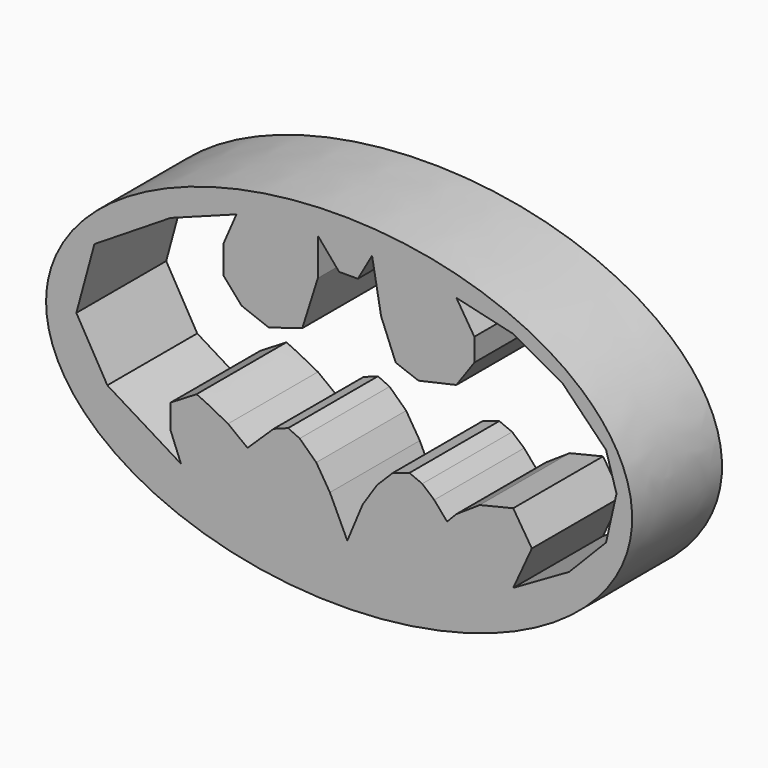
from build123d import *

# Parameters (mm, degrees)
F1_DEPTH = 25.4


with BuildPart() as f1:
    # F0 (on Front) → F1 (new body)
    with BuildSketch(Plane.XZ):
        with BuildLine():
            add(Edge.make_bspline(
                [(-66.2678331137, 0), (-66.2678331137, -67.3857780636), (33.1339165568, -33.6928890318), (132.5356662273, 0), (33.1339165568, 33.6928890318), (-66.2678331137, 67.3857780636), (-66.2678331137, 0)],
                knots=[0, 0, 0, 2.0943951024, 2.0943951024, 4.1887902048, 4.1887902048, 6.2831853072, 6.2831853072, 6.2831853072], degree=2, weights=[1, 0.5, 1, 0.5, 1, 0.5, 1]))
        make_face()
        with BuildLine():
            add(Edge.make_bspline(
                [(-38.1069518626, 25.8426479995), (-33.1428280721, 27.69202739), (-28.1787042816, 29.5414067805), (-23.2145804912, 31.390786171)],
                knots=[0, 0, 0, 0, 15.892279957, 15.892279957, 15.892279957, 15.892279957], degree=3))
            add(Edge.make_bspline(
                [(-23.2145804912, 31.390786171), (-24.1879379998, 29.152063032), (-25.1612955083, 26.913339893), (-26.1346530169, 24.6746167541)],
                knots=[0, 0, 0, 0, 7.3235070282, 7.3235070282, 7.3235070282, 7.3235070282], degree=3))
            add(Edge.make_bspline(
                [(-26.1346530169, 24.6746167541), (-26.1346530169, 22.5332298627), (-26.1346530169, 20.3918429712), (-26.1346530169, 18.2504560798)],
                knots=[0, 0, 0, 0, 6.4241606742, 6.4241606742, 6.4241606742, 6.4241606742], degree=3))
            add(Edge.make_bspline(
                [(-26.1346530169, 18.2504560798), (-24.7719523807, 16.6930838798), (-23.4092517445, 15.1357116799), (-22.0465511084, 13.5783394799)],
                knots=[0, 0, 0, 0, 6.2081600123, 6.2081600123, 6.2081600123, 6.2081600123], degree=3))
            add(Edge.make_bspline(
                [(-22.0465511084, 13.5783394799), (-20.0024998436, 12.7996532246), (-17.9584485789, 12.0209669694), (-15.9143973142, 11.2422807142)],
                knots=[0, 0, 0, 0, 6.5620485149, 6.5620485149, 6.5620485149, 6.5620485149], degree=3))
            add(Edge.make_bspline(
                [(-15.9143973142, 11.2422807142), (-13.3836676056, 12.0209669694), (-10.852937897, 12.7996532246), (-8.3222081885, 13.5783394799)],
                knots=[0, 0, 0, 0, 7.9434568216, 7.9434568216, 7.9434568216, 7.9434568216], degree=3))
            add(Edge.make_bspline(
                [(-8.3222081885, 13.5783394799), (-7.1541789609, 17.2770985713), (-5.9861497333, 20.9758576627), (-4.8181205057, 24.6746167541)],
                knots=[0, 0, 0, 0, 11.6364083735, 11.6364083735, 11.6364083735, 11.6364083735], degree=3))
            add(Edge.make_bspline(
                [(-4.8181205057, 24.6746167541), (-4.8181205057, 27.4973536531), (-4.8181205057, 30.3200905522), (-4.8181205057, 33.1428274512)],
                knots=[0, 0, 0, 0, 8.4682106972, 8.4682106972, 8.4682106972, 8.4682106972], degree=3))
            add(Edge.make_bspline(
                [(-4.8181205057, 33.1428274512), (-3.2120803371, 31.2610028519), (-1.6060401686, 29.3791782525), (0, 27.4973536531)],
                knots=[0, 0, 0, 0, 7.4219714101, 7.4219714101, 7.4219714101, 7.4219714101], degree=3))
            add(Edge.make_bspline(
                [(4.2341067456, 27.4973536531), (2.8227378304, 27.4973536531), (1.4113689152, 27.4973536531), (0, 27.4973536531)],
                knots=[0, 0, 0, 0, 4.2341067456, 4.2341067456, 4.2341067456, 4.2341067456], degree=3))
            add(Edge.make_bspline(
                [(4.2341067456, 27.4973536531), (5.3048000361, 29.3791782525), (6.3754933265, 31.2610028519), (7.446186617, 33.1428274512)],
                knots=[0, 0, 0, 0, 6.4952930269, 6.4952930269, 6.4952930269, 6.4952930269], degree=3))
            add(Edge.make_bspline(
                [(7.446186617, 33.1428274512), (8.1275366247, 29.3467330436), (8.8088866323, 25.550638636), (9.49023664, 21.7545442283)],
                knots=[0, 0, 0, 0, 11.570269455, 11.570269455, 11.570269455, 11.570269455], degree=3))
            add(Edge.make_bspline(
                [(9.49023664, 21.7545442283), (10.5910257747, 19.0358640005), (11.6918149094, 16.3171837727), (12.7926040441, 13.5985035449)],
                knots=[0, 0, 0, 0, 8.7992403138, 8.7992403138, 8.7992403138, 8.7992403138], degree=3))
            add(Edge.make_bspline(
                [(12.7926040441, 13.5985035449), (14.5068193475, 12.9556724181), (16.221034651, 12.3128412912), (17.9352499545, 11.6700101644)],
                knots=[0, 0, 0, 0, 5.4923486487, 5.4923486487, 5.4923486487, 5.4923486487], degree=3))
            add(Edge.make_bspline(
                [(17.9352499545, 11.6700101644), (20.7922750463, 12.3128412912), (23.6493001382, 12.9556724181), (26.50632523, 13.5985035449)],
                knots=[0, 0, 0, 0, 8.7853524743, 8.7853524743, 8.7853524743, 8.7853524743], degree=3))
            add(Edge.make_bspline(
                [(26.50632523, 13.5985035449), (27.8634124746, 15.5269963046), (29.2204997192, 17.4554890643), (30.5775869638, 19.3839818239)],
                knots=[0, 0, 0, 0, 7.0743855579, 7.0743855579, 7.0743855579, 7.0743855579], degree=3))
            add(Edge.make_bspline(
                [(30.5775869638, 19.3839818239), (30.5775869638, 21.0981971274), (30.5775869638, 22.8124124308), (30.5775869638, 24.5266277343)],
                knots=[0, 0, 0, 0, 5.1426459104, 5.1426459104, 5.1426459104, 5.1426459104], degree=3))
            add(Edge.make_bspline(
                [(30.5775869638, 24.5266277343), (29.2204997192, 26.6693979502), (27.8634124746, 28.812168166), (26.50632523, 30.9549383819)],
                knots=[0, 0, 0, 0, 7.6090965224, 7.6090965224, 7.6090965224, 7.6090965224], degree=3))
            add(Edge.make_bspline(
                [(26.50632523, 30.9549383819), (30.7918662826, 29.9549791962), (35.0774073352, 28.9550200105), (39.3629483879, 27.9550608248)],
                knots=[0, 0, 0, 0, 13.2019704734, 13.2019704734, 13.2019704734, 13.2019704734], degree=3))
            add(Edge.make_bspline(
                [(39.3629483879, 27.9550608248), (43.0770814419, 25.8882219593), (46.7912144959, 23.8213830938), (50.5053475499, 21.7545442283)],
                knots=[0, 0, 0, 0, 12.7514495313, 12.7514495313, 12.7514495313, 12.7514495313], degree=3))
            add(Edge.make_bspline(
                [(50.5053475499, 21.7545442283), (53.7909269333, 18.3930328737), (57.0765063167, 15.031521519), (60.3620857, 11.6700101644)],
                knots=[0, 0, 0, 0, 14.1015287911, 14.1015287911, 14.1015287911, 14.1015287911], degree=3))
            add(Edge.make_bspline(
                [(60.3620857, 11.6700101644), (61.1477668087, 9.0272611318), (61.9334479173, 6.3845120991), (62.7191290259, 3.7417630665)],
                knots=[0, 0, 0, 0, 8.2712003533, 8.2712003533, 8.2712003533, 8.2712003533], degree=3))
            add(Edge.make_bspline(
                [(62.7191290259, 3.7417630665), (61.9334479173, 0.2419063821), (61.1477668087, -3.2579503022), (60.3620857, -6.7578069866)],
                knots=[0, 0, 0, 0, 10.7608840036, 10.7608840036, 10.7608840036, 10.7608840036], degree=3))
            add(Edge.make_bspline(
                [(60.3620857, -6.7578069866), (57.57648622, -9.6148330097), (54.7908867399, -12.4718590329), (52.0052872598, -15.3288850561)],
                knots=[0, 0, 0, 0, 11.9707752232, 11.9707752232, 11.9707752232, 11.9707752232], degree=3))
            add(Edge.make_bspline(
                [(52.0052872598, -15.3288850561), (47.7911743025, -17.7573567877), (43.5770613452, -20.1858285194), (39.3629483879, -22.614300251)],
                knots=[0, 0, 0, 0, 14.5912990071, 14.5912990071, 14.5912990071, 14.5912990071], degree=3))
            add(Edge.make_bspline(
                [(39.3629483879, -22.614300251), (40.767652707, -19.542997703), (42.1723570261, -16.4716951549), (43.5770613452, -13.4003926069)],
                knots=[0, 0, 0, 0, 10.1318725857, 10.1318725857, 10.1318725857, 10.1318725857], degree=3))
            add(Edge.make_bspline(
                [(43.5770613452, -13.4003926069), (42.1723570261, -11.1861974001), (40.767652707, -8.9720021933), (39.3629483879, -6.7578069866)],
                knots=[0, 0, 0, 0, 7.8665552652, 7.8665552652, 7.8665552652, 7.8665552652], degree=3))
            add(Edge.make_bspline(
                [(39.3629483879, -6.7578069866), (36.8456294139, -7.3634053891), (34.32831044, -7.9690037916), (31.810991466, -8.5746021941)],
                knots=[0, 0, 0, 0, 7.7674190163, 7.7674190163, 7.7674190163, 7.7674190163], degree=3))
            add(Edge.make_bspline(
                [(31.810991466, -8.5746021941), (30.0320349634, -9.7605735064), (28.2530784607, -10.9465448186), (26.474121958, -12.1325161308)],
                knots=[0, 0, 0, 0, 6.4141194038, 6.4141194038, 6.4141194038, 6.4141194038], degree=3))
            add(Edge.make_bspline(
                [(26.474121958, -12.1325161308), (25.7875068734, -12.8503410767), (25.1008917888, -13.5681660225), (24.4142767042, -14.2859909683)],
                knots=[0, 0, 0, 0, 2.9800027426, 2.9800027426, 2.9800027426, 2.9800027426], degree=3))
            add(Edge.make_bspline(
                [(24.4142767042, -14.2859909683), (23.4467734893, -13.1624390682), (22.4792702744, -12.038887168), (21.5117670596, -10.9153352678)],
                knots=[0, 0, 0, 0, 4.4481324271, 4.4481324271, 4.4481324271, 4.4481324271], degree=3))
            add(Edge.make_bspline(
                [(21.5117670596, -10.9153352678), (20.6066835672, -10.1350909099), (19.7016000748, -9.354846552), (18.7965165824, -8.5746021941)],
                knots=[0, 0, 0, 0, 3.5849151281, 3.5849151281, 3.5849151281, 3.5849151281], degree=3))
            add(Edge.make_bspline(
                [(18.7965165824, -8.5746021941), (17.8290139884, -8.1708699258), (16.8615113944, -7.7671376574), (15.8940088004, -7.3634053891)],
                knots=[0, 0, 0, 0, 3.1450833256, 3.1450833256, 3.1450833256, 3.1450833256], degree=3))
            add(Edge.make_bspline(
                [(15.8940088004, -7.3634053891), (14.6456177657, -7.7671376574), (13.397226731, -8.1708699258), (12.1488356963, -8.5746021941)],
                knots=[0, 0, 0, 0, 3.9361553933, 3.9361553933, 3.9361553933, 3.9361553933], degree=3))
            add(Edge.make_bspline(
                [(12.1488356963, -8.5746021941), (10.9628643841, -9.7605735064), (9.7768930718, -10.9465448186), (8.5909217596, -12.1325161308)],
                knots=[0, 0, 0, 0, 5.031650143, 5.031650143, 5.031650143, 5.031650143], degree=3))
            add(Edge.make_bspline(
                [(8.5909217596, -12.1325161308), (7.4985795654, -13.7866344303), (6.4062373713, -15.4407527298), (5.3138951771, -17.0948710293)],
                knots=[0, 0, 0, 0, 5.9467528417, 5.9467528417, 5.9467528417, 5.9467528417], degree=3))
            add(Edge.make_bspline(
                [(5.3138951771, -17.0948710293), (4.1591336097, -19.872540608), (3.0043720423, -22.6502101868), (1.8496104749, -25.4278797656)],
                knots=[0, 0, 0, 0, 9.0244281314, 9.0244281314, 9.0244281314, 9.0244281314], degree=3))
            add(Edge.make_bspline(
                [(1.8496104749, -25.4278797656), (0.5388003774, -22.6502101868), (-0.7720097201, -19.872540608), (-2.0828198176, -17.0948710293)],
                knots=[0, 0, 0, 0, 9.214284704, 9.214284704, 9.214284704, 9.214284704], degree=3))
            add(Edge.make_bspline(
                [(-2.0828198176, -17.0948710293), (-3.1127426773, -15.4407527298), (-4.1426655371, -13.7866344303), (-5.1725883968, -12.1325161308)],
                knots=[0, 0, 0, 0, 5.845651034, 5.845651034, 5.845651034, 5.845651034], degree=3))
            add(Edge.make_bspline(
                [(-5.1725883968, -12.1325161308), (-6.4209789659, -10.9465448186), (-7.6693695349, -9.7605735064), (-8.9177601039, -8.5746021941)],
                knots=[0, 0, 0, 0, 5.1657586758, 5.1657586758, 5.1657586758, 5.1657586758], degree=3))
            add(Edge.make_bspline(
                [(-8.9177601039, -8.5746021941), (-9.7916334247, -8.1708699258), (-10.6655067454, -7.7671376574), (-11.5393800661, -7.3634053891)],
                knots=[0, 0, 0, 0, 2.8878865848, 2.8878865848, 2.8878865848, 2.8878865848], degree=3))
            add(Edge.make_bspline(
                [(-11.5393800661, -7.3634053891), (-12.6317227259, -7.7671376574), (-13.7240653858, -8.1708699258), (-14.8164080456, -8.5746021941)],
                knots=[0, 0, 0, 0, 3.4936957622, 3.4936957622, 3.4936957622, 3.4936957622], degree=3))
            add(Edge.make_bspline(
                [(-14.8164080456, -8.5746021941), (-16.7826227844, -10.4783984522), (-18.7488375232, -12.3821947103), (-20.7150522619, -14.2859909683)],
                knots=[0, 0, 0, 0, 8.2106007893, 8.2106007893, 8.2106007893, 8.2106007893], degree=3))
            add(Edge.make_bspline(
                [(-20.7150522619, -14.2859909683), (-22.1819126358, -13.1624390682), (-23.6487730096, -12.038887168), (-25.1156333834, -10.9153352678)],
                knots=[0, 0, 0, 0, 5.5431429765, 5.5431429765, 5.5431429765, 5.5431429765], degree=3))
            add(Edge.make_bspline(
                [(-25.1156333834, -10.9153352678), (-28.2862470927, -9.2344051743), (-31.456860802, -7.5534750809), (-32.2668068111, -7.3634053891)],
                knots=[0, 0, 0, 0, 0.8394649966, 0.8394649966, 0.8394649966, 0.8394649966], degree=3))
            add(Edge.make_bspline(
                [(-32.2668068111, -7.3634053891), (-34.2135218283, -8.5473820153), (-36.1602368454, -9.7313586416), (-38.1069518626, -10.9153352678)],
                knots=[0, 0, 0, 0, 6.8354590252, 6.8354590252, 6.8354590252, 6.8354590252], degree=3))
            add(Edge.make_bspline(
                [(-38.1069518626, -10.9153352678), (-38.1069518626, -12.7674552302), (-38.1069518626, -14.6195751925), (-38.1069518626, -16.4716951549)],
                knots=[0, 0, 0, 0, 5.5563598871, 5.5563598871, 5.5563598871, 5.5563598871], degree=3))
            add(Edge.make_bspline(
                [(-38.1069518626, -16.4716951549), (-37.3282656074, -18.4273160994), (-36.5495793521, -20.3829370439), (-35.7708930969, -22.3385579884)],
                knots=[0, 0, 0, 0, 6.3148436294, 6.3148436294, 6.3148436294, 6.3148436294], degree=3))
            add(Edge.make_bspline(
                [(-35.7708930969, -22.3385579884), (-41.3190325101, -18.9365440359), (-46.8671719233, -15.5345300833), (-52.4153113365, -12.1325161308)],
                knots=[0, 0, 0, 0, 19.5243424712, 19.5243424712, 19.5243424712, 19.5243424712], degree=3))
            add(Edge.make_bspline(
                [(-52.4153113365, -12.1325161308), (-54.7513701022, -8.0883440872), (-57.0874288678, -4.0441720436), (-59.4234876335, 0)],
                knots=[0, 0, 0, 0, 14.0111556509, 14.0111556509, 14.0111556509, 14.0111556509], degree=3))
            add(Edge.make_bspline(
                [(-59.4234876335, 0), (-58.0607863764, 5.0127919142), (-56.6980851193, 10.0255838285), (-55.3353838623, 15.0383757427)],
                knots=[0, 0, 0, 0, 15.5841373654, 15.5841373654, 15.5841373654, 15.5841373654], degree=3))
            add(Edge.make_bspline(
                [(-55.3353838623, 15.0383757427), (-49.5925731957, 18.6397998283), (-43.8497625291, 22.2412239139), (-38.1069518626, 25.8426479995)],
                knots=[0, 0, 0, 0, 20.3359575178, 20.3359575178, 20.3359575178, 20.3359575178], degree=3))
        make_face(mode=Mode.SUBTRACT)
    extrude(amount=F1_DEPTH)


solid = f1.part
